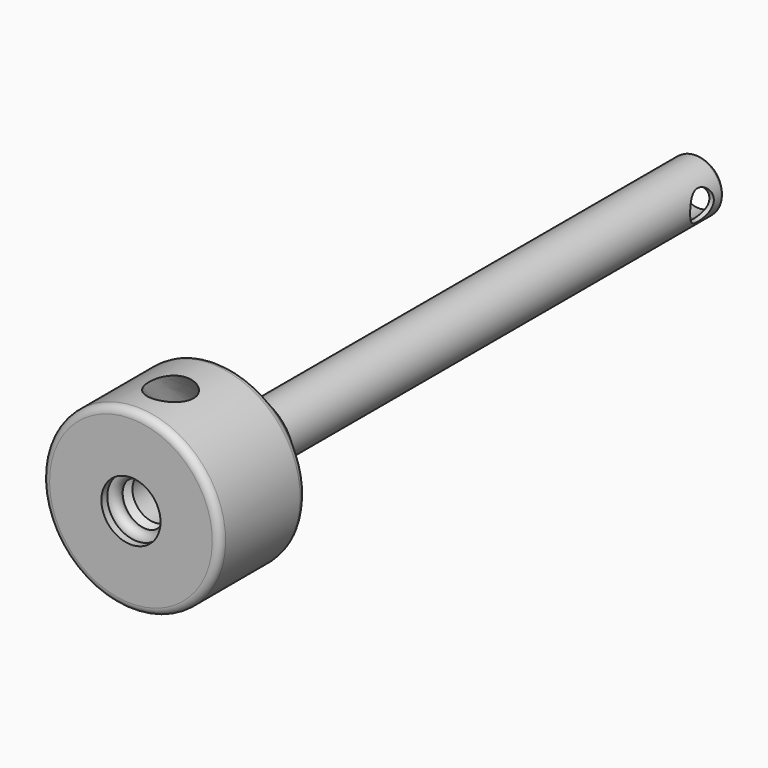
from build123d import *

# Parameters (mm, degrees)
F3_R     = 0.1
F4_R     = 0.25
F6_R     = 0.75
F8_R     = 0.5
F9_DEPTH = 2.5


with BuildPart() as f2:
    # F0 (on Right) → F2 (revolve)
    with BuildSketch(Plane.YZ):
        with BuildLine():
            Line((11.5, 3), (8, 3))
            Line((8, 3), (8, 1))
            Line((8, 1), (8.25, 1))
            ThreePointArc((8.25, 1), (8.5, 0.75), (8.75, 1))
            Line((8.75, 1), (9, 0.75))
            Line((9, 0.75), (32, 0.75))
            Line((32, 0.75), (31.85, 0.9))
            Line((31.85, 0.9), (13, 0.9))
            Line((13, 0.9), (13, 1.5))
            Line((13, 1.5), (11.5, 3))
        make_face()
    revolve(axis=Axis((0, 17.771827057, 0), (0, 1, 0)))

    # F3
    f3_edges = [f2.edges().sort_by_distance(p)[0] for p in [
        (0, 31.85, -0.9),
        (0, 13, -0.9),
    ]]
    fillet(f3_edges, radius=F3_R)

    # F4
    f4_edges = [f2.edges().sort_by_distance(p)[0] for p in [
        (0, 13, -1.5),
        (0, 11.5, -3),
        (0, 8, -3),
    ]]
    fillet(f4_edges, radius=F4_R)

    # F7: sweep along a path in F5
    with BuildLine(Plane.YZ) as f7_path:
        Line((3.6301804626, 10), (11.391852051, 0.75))
    # F6 (on Top) → F7 (sweep, cut)
    with BuildSketch(Plane.XY):
        with Locations((0, 12.141852051)):
            Circle(F6_R)
    sweep(path=f7_path.line, mode=Mode.SUBTRACT)

    # F8 (on Right) → F9 (cut, symmetric)
    with BuildSketch(Plane.YZ):
        with Locations((31, 0)):
            Circle(F8_R)
    extrude(amount=F9_DEPTH, both=True, mode=Mode.SUBTRACT)


solid = f2.part
